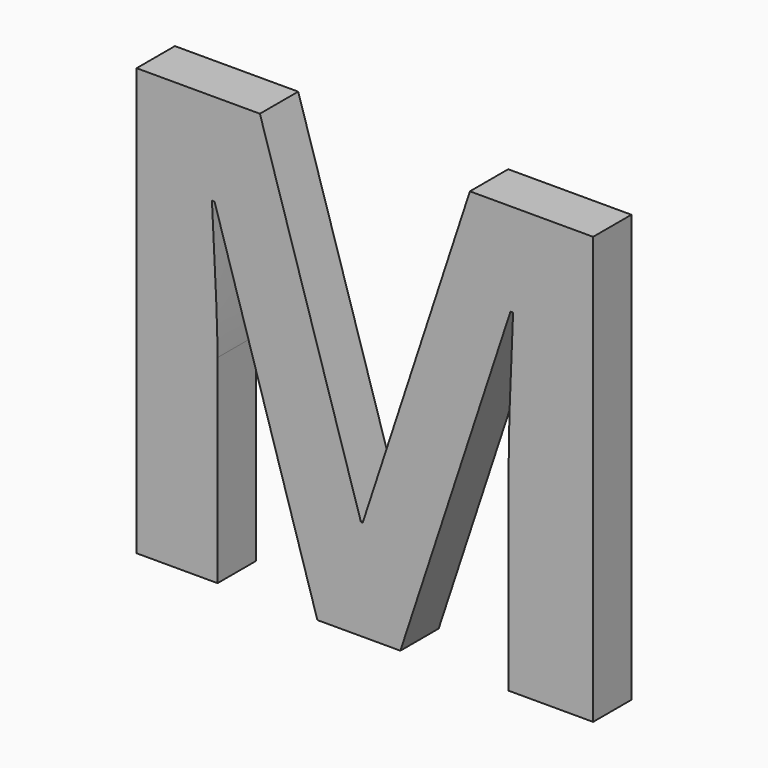
from build123d import *

# Parameters (mm, degrees)
F0_TEXT_SIZE = 62.5
F1_DEPTH     = 5


# Not quite as in the source:
# - Text() gives the source's letters only with a copy of the font that has no kerning and outlines rounded to 1/6400 em; it was checked with that copy


with BuildPart() as f1:
    # F0 (on Front) → F1 (new body)
    with BuildSketch(Plane.XZ):
        with Locations((-65.1766289339, 15.896738187)):
            Text('M', F0_TEXT_SIZE, font='Open Sans', font_style=FontStyle.BOLD, text_align=(TextAlign.LEFT, TextAlign.BOTTOM))
    extrude(amount=F1_DEPTH)


solid = f1.part
